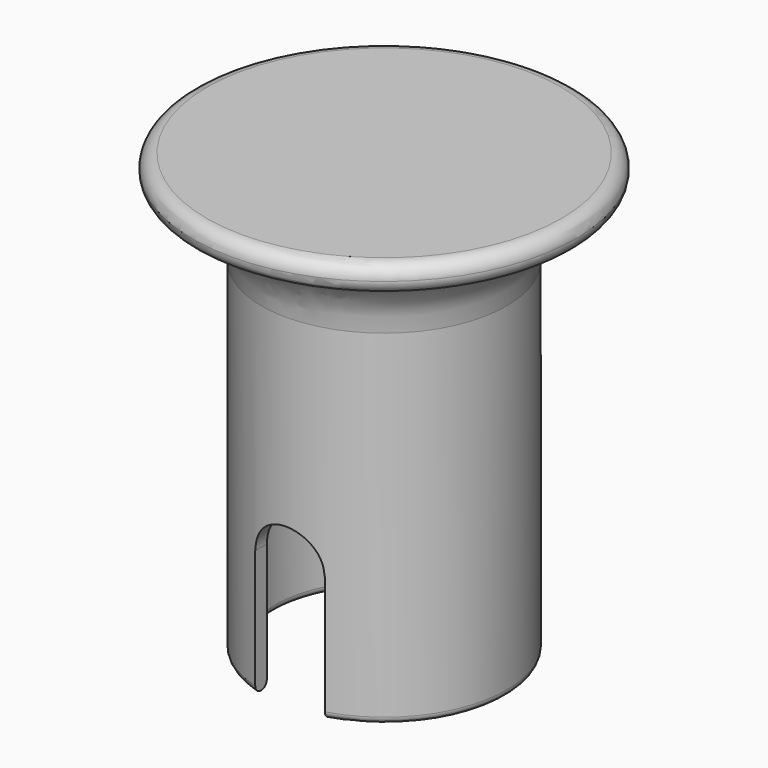
from build123d import *

# Parameters (mm, degrees)
F2_R     = 0.99999
F3_R     = 5
F4_R     = 0.49999
F5_R     = 2.4176485657
F6_DEPTH = 89.5
F7_R     = 2
F9_DEPTH = 39.1


# Not quite as in the source:
# - a fillet or chamfer is up to 0.001 mm smaller than in the source, because OpenCascade refuses the exact size


with BuildPart() as f1:
    # F0 (on Right) → F1 (revolve)
    with BuildSketch(Plane.YZ):
        Polygon((-35.6084575608, -62.0439687319), (-34.6084575608, -62.0439687319), (-34.6084575608, -32.0439687319), (-26.7034575608, -32.0439687319), (-26.7034575608, -30.0439687319), (-40.6084575608, -30.0439687319), (-40.6084575608, -32.0439687319), (-35.6084575608, -32.0439687319), align=None)
    revolve(axis=Axis((0, -26.7034575608, -31.0439687319), (0, 0, 1)))

    # F2 (radius 1 in the source; OpenCascade refuses exactly that, so slightly less here)
    f2_edges = [f1.edges().sort_by_distance(p)[0] for p in [
        (0, -12.798458, -32.043969),
        (0, -12.798458, -30.043969),
    ]]
    fillet(f2_edges, radius=F2_R)

    # F3
    f3_edges = [f1.edges().sort_by_distance(p)[0] for p in [
        (0, -17.798458, -32.043969),
    ]]
    fillet(f3_edges, radius=F3_R)

    # F4 (radius 0.5 in the source; OpenCascade refuses exactly that, so slightly less here)
    f4_edges = [f1.edges().sort_by_distance(p)[0] for p in [
        (0, -18.798458, -62.043969),
        (0, -17.798458, -62.043969),
    ]]
    fillet(f4_edges, radius=F4_R)

    # F5 (on Front) → F6 (cut)
    with BuildSketch(Plane.XZ):
        with Locations((0, -61.6349689662)):
            Circle(F5_R)
    extrude(amount=F6_DEPTH, mode=Mode.SUBTRACT)

    # F7
    f7_edges = [f1.edges().sort_by_distance(p)[0] for p in [
        (0, -18.798458, -32.043969),
    ]]
    fillet(f7_edges, radius=F7_R)

    # F8 (on Front) → F9 (cut)
    with BuildSketch(Plane.XZ):
        with BuildLine():
            Line((-2.5493614376, -52.8711415827), (-2.5493614376, -62.0828643441))
            Line((-2.5493614376, -62.0828643441), (2.5154370815, -62.0695389807))
            Line((2.5154370815, -62.0695389807), (2.5154370815, -52.8711415827))
            Line((2.5154370815, -52.8711415827), (2.4968570896, -52.8711415827))
            ThreePointArc((2.4968570896, -52.8711415827), (-0.0169621781, -55.3849608503), (-2.5307814457, -52.8711415827))
            Line((-2.5307814457, -52.8711415827), (-2.5493614376, -52.8711415827))
        make_face()
        with BuildLine():
            ThreePointArc((2.4968570896, -52.8711415827), (-0.0169621781, -50.3573223151), (-2.5307814457, -52.8711415827))
            Line((-2.5307814457, -52.8711415827), (2.4968570896, -52.8711415827))
        make_face()
        with BuildLine():
            Line((2.4968570896, -52.8711415827), (-2.5307814457, -52.8711415827))
            ThreePointArc((-2.5307814457, -52.8711415827), (-0.0169621781, -55.3849608503), (2.4968570896, -52.8711415827))
        make_face()
    extrude(amount=F9_DEPTH, mode=Mode.SUBTRACT)


solid = f1.part
